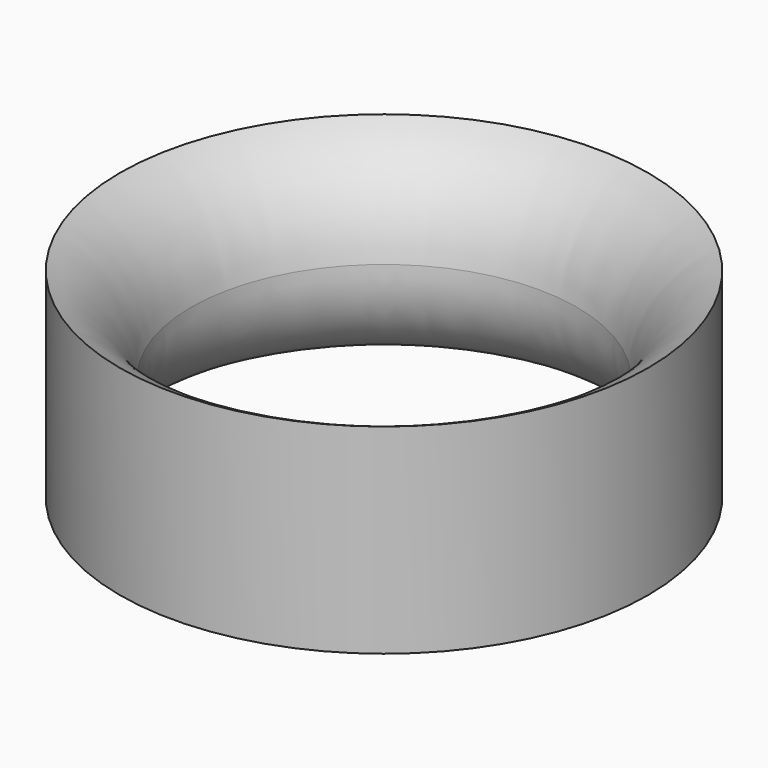
from build123d import *

# Parameters (mm, degrees)
F0_R     = 11
F0_R_2   = 8
F1_DEPTH = 8.33
F2_R     = 11.5325347533
F2_R_2   = 11
F3_DEPTH = 25


# Not quite as in the source:
# - a fillet or chamfer that OpenCascade refuses, or shapes differently, is made with other operations: its cross-section is extruded or revolved along the edge and cut away or added


with BuildPart() as f1:
    # F0 (on Top) → F1 (new body)
    with BuildSketch(Plane.XY):
        Circle(F0_R)
        Circle(F0_R_2, mode=Mode.SUBTRACT)
    extrude(amount=F1_DEPTH)

    # F2 (on face) → F3 (cut)
    with BuildSketch(Plane.XY.offset(8.33)):
        Circle(F2_R)
        Circle(F2_R_2, mode=Mode.SUBTRACT)
    extrude(amount=-F3_DEPTH, mode=Mode.SUBTRACT)

    # F4: fillet of radius 5 on 1 edges, made by hand

    # F4_s1 → F4_t2 (revolve, cut)
    with BuildSketch(Plane.XZ):
        with BuildLine():
            ThreePointArc((8, 3.747424305), (8.8166998673, 6.4860370926), (11, 8.33))
            Line((11, 8.33), (8, 8.33))
            Line((8, 8.33), (8, 3.747424305))
        make_face()
    revolve(axis=Axis((0, 0, 8.33), (0, 0, 1)), mode=Mode.SUBTRACT)

    # F5: fillet of radius 4 on 1 edges, made by hand

    # F5_s1 → F5_t2 (revolve, cut)
    with BuildSketch(Plane.XZ):
        with BuildLine():
            ThreePointArc((11, 0), (8.6975924738, 1.6252394507), (8.0383219615, 4.3652843555))
            Line((8.0383219615, 4.3652843555), (7.6413877184, 4.4147131595))
            ThreePointArc((7.6413877184, 4.4147131595), (7.6, 3.747424305), (7.6, 0))
            Line((7.6, 0), (8, -0.4))
            ThreePointArc((8, -0.4), (9.5, -0.4), (10.8992335608, -0.3870996315))
            Line((10.8992335608, -0.3870996315), (11, 0))
        make_face()
    revolve(axis=Axis((0, 0, 0), (0, 0, 1)), mode=Mode.SUBTRACT)


solid = f1.part
